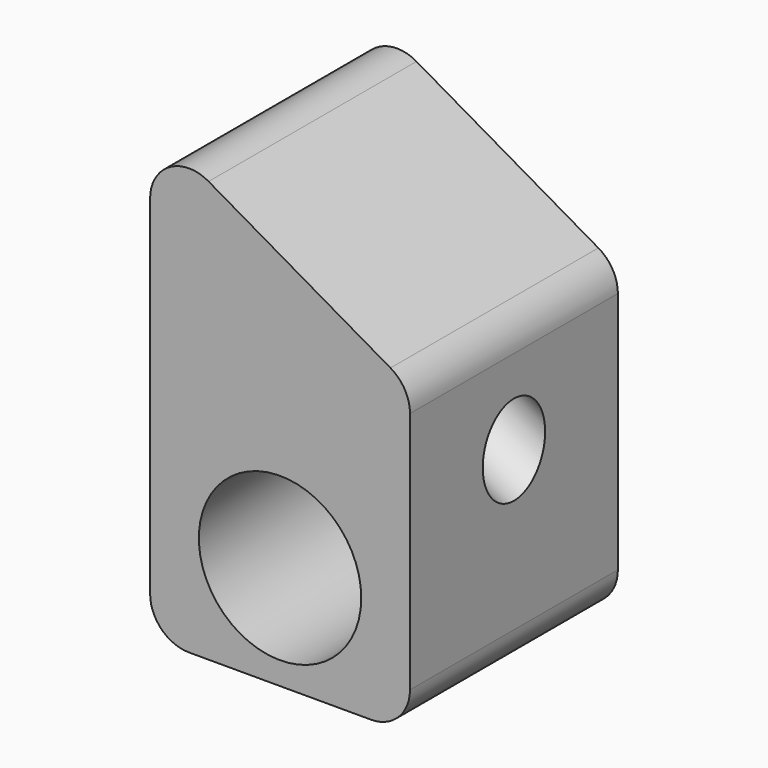
from build123d import *

# Parameters (mm, degrees)
F1_DEPTH       = 20
F5_D           = 6.6
F5_CBORE_D     = 12.5
F5_CBORE_DEPTH = 12
F7_T1_DEPTH    = 45.9807621135
F7_T3_DEPTH    = 28.6602540378
F7_T5_DEPTH    = 35


# Not quite as in the source:
# - a fillet or chamfer that OpenCascade refuses, or shapes differently, is made with other operations: its cross-section is extruded or revolved along the edge and cut away or added


with BuildPart() as f1:
    # F0 (on Front) → F1 (new body)
    with BuildSketch(Plane.XZ):
        Polygon((-10, -20), (10, -20), (10, 3.4529946162), (-10, 15), align=None)
    extrude(amount=F1_DEPTH)

    # F5 (through all)
    with Locations(Plane.XZ.offset(20)):
        with Locations((0, -12)):
            CounterBoreHole(F5_D / 2, F5_CBORE_D / 2, F5_CBORE_DEPTH)

    # F3 (on offset) → F6 (revolve, cut)
    with BuildSketch(Plane.XZ.offset(10)):
        Polygon((-10.3968404344, 10.6191993773), (-10.3968404344, 6.9818926814), (13.3675798804, -6.7385017846), (13.3675798804, -3.2744001694), (2.5, 3), (0, 3), (0.8023552889, 4.1533407117), align=None)
    revolve(axis=Axis((1.485369723, -10, 0.1216954484), (-0.8660254038, 0, 0.5)), mode=Mode.SUBTRACT)

    # F7: fillet of radius 3 on 4 edges, made by hand

    # F7_s2 → F7_t1 (cut)
    with BuildSketch(Plane.XZ.offset(-12.9903810568)):
        with BuildLine():
            ThreePointArc((-5.5, 12.4019237886), (-8.5, 12.4019237886), (-10, 9.8038475773))
            Line((-10, 9.8038475773), (-10, 15))
            Line((-10, 15), (-5.5, 12.4019237886))
        make_face()
    extrude(amount=F7_T1_DEPTH, mode=Mode.SUBTRACT)

    # F7_s4 → F7_t3 (cut)
    with BuildSketch(Plane.XZ.offset(-4.3301270189)):
        with BuildLine():
            ThreePointArc((8.5, 4.31902002), (9.5980762114, 3.2209438086), (10, 1.7209438086))
            Line((10, 1.7209438086), (10, 3.4529946162))
            Line((10, 3.4529946162), (8.5, 4.31902002))
        make_face()
    extrude(amount=F7_T3_DEPTH, mode=Mode.SUBTRACT)

    # F7_s6 → F7_t5 (cut)
    with BuildSketch(Plane.XZ.offset(-7.5)):
        with BuildLine():
            ThreePointArc((10, -17), (9.1213203436, -19.1213203436), (7, -20))
            Line((7, -20), (10, -20))
            Line((10, -20), (10, -17))
        make_face()
        with BuildLine():
            ThreePointArc((-10, -17), (-9.1213203436, -19.1213203436), (-7, -20))
            Line((-7, -20), (-10, -20))
            Line((-10, -20), (-10, -17))
        make_face()
    extrude(amount=F7_T5_DEPTH, mode=Mode.SUBTRACT)


solid = f1.part
